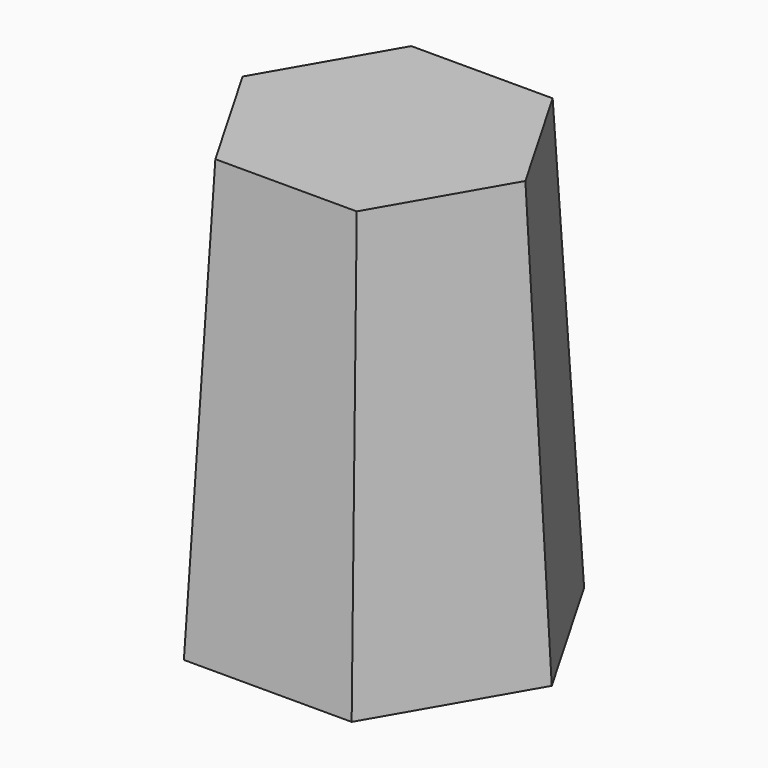
from build123d import *

# Parameters (mm, degrees)
F1_DEPTH = 76.2
F1_TAPER = 3


with BuildPart() as f1:
    # F0 (on Top) → F1 (new body)
    with BuildSketch(Plane.XY):
        Polygon((-43.9940905122, 25.4), (-29.3293936748, 0), (0, 0), (14.6646968374, 25.4), (0, 50.8), (-29.3293936748, 50.8), align=None)
    extrude(amount=F1_DEPTH, taper=F1_TAPER)


solid = f1.part
